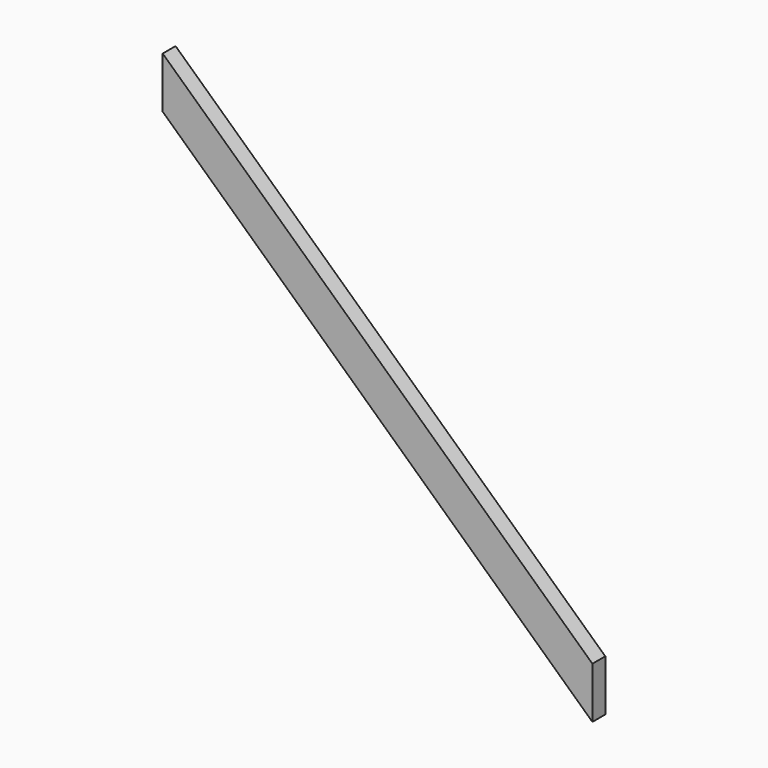
from build123d import *

# Parameters (mm, degrees)
F1_DEPTH = 38.1


# Not quite as in the source:
# - a feature names something its author has since deleted; it is built from what else it names


with BuildPart() as f1:
    # F0 (on Front) → F1 (new body)
    with BuildSketch(Plane.XZ):
        Polygon((1015.9991338121, -939.7991987762), (0, 0), (0, -121.1007599326), (1015.9991338121, -1060.8999587088), align=None)
    extrude(amount=-F1_DEPTH)


solid = f1.part
